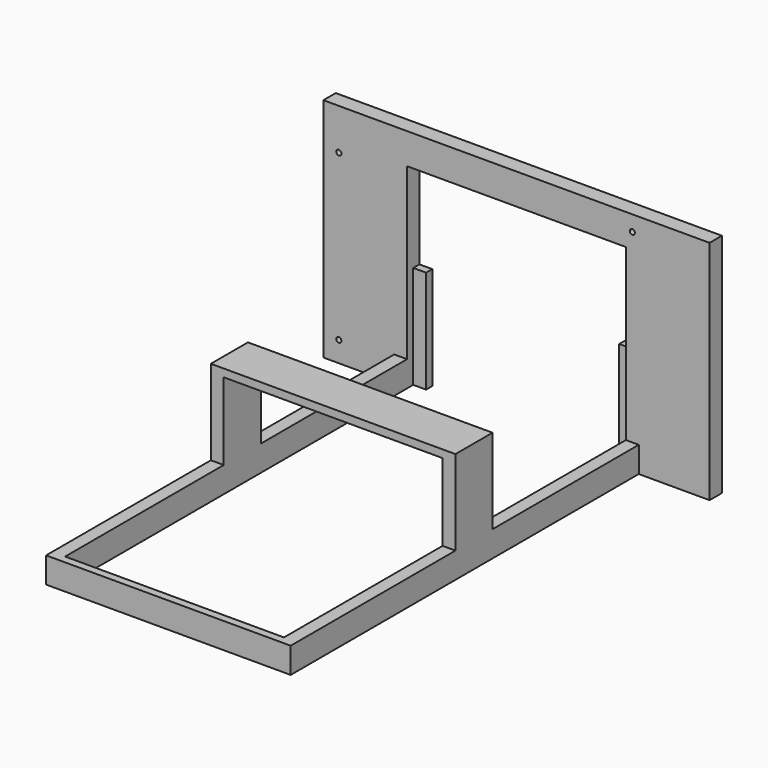
from build123d import *

# Parameters (mm, degrees)
F0_W     = 5
F0_H     = 3
F0_H_2   = 30
F1_DEPTH = 6
F0_H_3   = 10
F2_DEPTH = 175
F3_DEPTH = 3
F4_START = 172
F0_W_2   = 75
F4_DEPTH = 3
F5_START = 77
F5_DEPTH = 18
F6_D     = 2


# Not quite as in the source:
# - a feature names something its author has since deleted; it is built from what else it names


with BuildPart() as f1:
    # F0 (on Front) → F1 (new body)
    with BuildSketch(Plane.XZ):
        Polygon((75, 48), (-75, 48), (-75, -40), (-47.5, -40), (-47.5, -30), (-47.5, 0), (-47.5, 3), (-42.5, 3), (-42.5, 36), (42.5, 36), (75, 36), align=None)
        Polygon((75, -40), (75, 36), (42.5, 36), (42.5, 3), (47.5, 3), (47.5, 0), (47.5, -30), (47.5, -40), align=None)
        with Locations((45, 1.5)):
            Rectangle(F0_W, F0_H)
        with Locations((45, -15)):
            Rectangle(F0_W, F0_H_2)
        with Locations((-45, 1.5)):
            Rectangle(F0_W, F0_H)
        with Locations((-45, -15)):
            Rectangle(F0_W, F0_H_2)
    extrude(amount=F1_DEPTH)

    # F0 (on Front) → F2 (join)
    with BuildSketch(Plane.XZ):
        with Locations((-45, -35)):
            Rectangle(F0_W, F0_H_3)
        with Locations((45, -35)):
            Rectangle(F0_W, F0_H_3)
    extrude(amount=F2_DEPTH)

    # F0 (on Front) → F3 (join)
    with BuildSketch(Plane.XZ):
        with Locations((-40, -15)):
            Rectangle(F0_W, F0_H_2)
        with Locations((-40, -35)):
            Rectangle(F0_W, F0_H_3)
        with Locations((40, -35)):
            Rectangle(F0_W, F0_H_3)
        with Locations((40, -15)):
            Rectangle(F0_W, F0_H_2)
    extrude(amount=F3_DEPTH)

    # F0 (on Front) → F4 (join)
    with BuildSketch(Plane.XZ.offset(F4_START)):
        with Locations((-40, -35)):
            Rectangle(F0_W, F0_H_3)
        with Locations((40, -35)):
            Rectangle(F0_W, F0_H_3)
        with Locations((0, -35)):
            Rectangle(F0_W_2, F0_H_3)
    extrude(amount=F4_DEPTH)

    # F0 (on Front) → F5 (join)
    with BuildSketch(Plane.XZ.offset(F5_START)):
        with Locations((-45, -15)):
            Rectangle(F0_W, F0_H_2)
        with Locations((45, -15)):
            Rectangle(F0_W, F0_H_2)
        Polygon((42.5, 0), (42.5, 3), (-42.5, 3), (-42.5, 0), (-37.5, 0), (37.5, 0), align=None)
        with Locations((45, 1.5)):
            Rectangle(F0_W, F0_H)
        with Locations((-45, 1.5)):
            Rectangle(F0_W, F0_H)
    extrude(amount=F5_DEPTH)

    # F6 (through all)
    with Locations(Plane(origin=(0, 0, 0), x_dir=(1, 0, 0), z_dir=(0, 1, 0))):
        with Locations((45, -42), (-69, -32), (-69, 32)):
            Hole(F6_D / 2)


solid = f1.part
